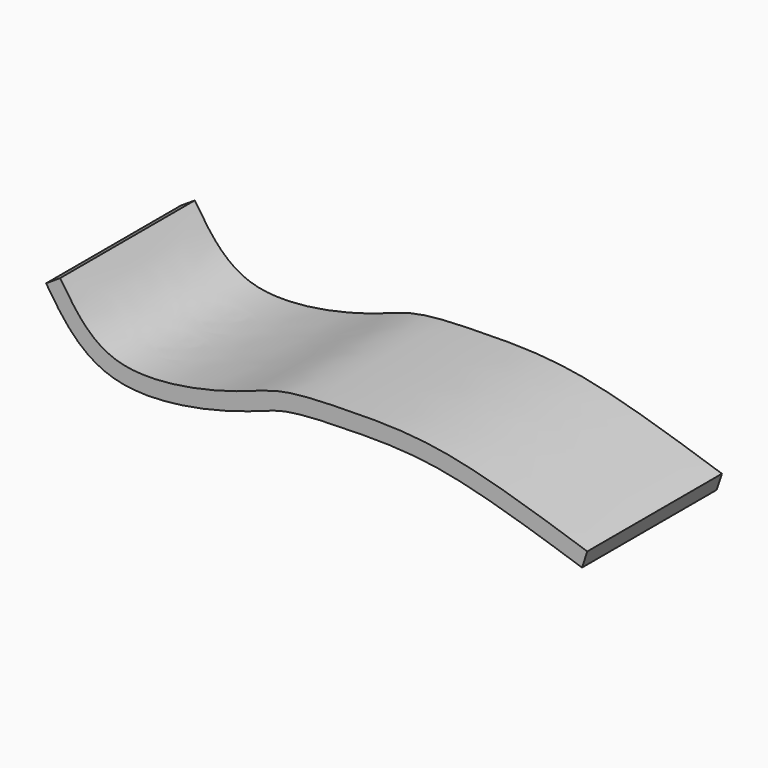
from build123d import *

# Parameters (mm, degrees)
F1_DEPTH = 30


# Not quite as in the source:
# - the dataset's text gives a spline's control points without its knots; the knots are read off the source's solid


with BuildPart() as f1:
    # F0 (on Front) → F1 (new body)
    with BuildSketch(Plane.XZ):
        with BuildLine():
            add(Edge.make_bspline(
                [(0, 0), (2.6760176861, -4.1090912765), (8.6109843066, -13.2223791643), (31.6156140644, -8.0154668369), (38.9230176312, -4.44082064), (51.783425309, -4.0415965154), (68.5152984785, -3.9207662334), (84.8401925941, -9.3146463612), (93.9818322659, -12.335119769)],
                knots=[0, 0, 0, 0, 0.1565314067, 0.3471608871, 0.4695561585, 0.6124947665, 0.7830042149, 1, 1, 1, 1], degree=3))
            Line((0, 0), (-2.5139018349, -1.6371614351))
            add(Edge.make_bspline(
                [(-2.5139018349, -1.6371614351), (-1.9796604679, -2.4575022542), (-0.8824950145, -4.1435116076), (0.9716962826, -6.681806788), (2.818494485, -8.6893851392), (4.557008715, -10.1358158216), (6.0060415743, -11.1092063701), (7.3415213838, -11.7998974719), (8.4850992129, -12.2638918131), (9.3820086025, -12.5650155809), (10.3070201286, -12.8131843436), (11.557238239, -13.0752296171), (13.1545045101, -13.2882162402), (15.1103366517, -13.3908370168), (17.7527257108, -13.3559807007), (21.0825413014, -13.0414284407), (24.9788204805, -12.3653086477), (28.0085066014, -11.6521555257), (30.2166637186, -11.0488210969), (31.7451800625, -10.5933469575), (33.119290683, -10.1496504012), (34.7509538884, -9.5877723837), (36.4769836834, -8.9563036794), (37.9277627865, -8.4589434042), (39.0494494043, -8.1389931547), (39.7663852968, -7.9682024182), (40.3766098683, -7.8468566795), (41.0225632514, -7.7333923842), (41.887025299, -7.6077797582), (43.0058157906, -7.482054254), (44.5913088845, -7.3455222102), (46.7249490736, -7.2266828348), (49.4553505745, -7.1438428112), (52.2981469692, -7.0863726415), (55.1415351216, -7.0513679222), (58.0217504556, -7.0809612374), (60.9631996142, -7.2074537938), (63.4895890714, -7.4223332941), (65.5709676375, -7.6772717752), (67.164506612, -7.9141125344), (68.7998566688, -8.2023954474), (71.0459002226, -8.6542298497), (73.959722197, -9.3354473137), (78.8117218745, -10.6357407606), (85.1614022918, -12.5803834941), (90.4076393103, -14.3136905098), (93.0406511874, -15.183659426)],
                knots=[0, 0, 0, 0, 0.03125, 0.0625, 0.09375, 0.109375, 0.125, 0.140625, 0.1484375, 0.15625, 0.1640625, 0.171875, 0.1875, 0.203125, 0.21875, 0.25, 0.28125, 0.3125, 0.328125, 0.34375, 0.359375, 0.375, 0.40625, 0.4375, 0.453125, 0.46875, 0.4765625, 0.484375, 0.5, 0.515625, 0.53125, 0.5625, 0.59375, 0.625, 0.65625, 0.6875, 0.71875, 0.75, 0.765625, 0.78125, 0.796875, 0.8125, 0.84375, 0.875, 0.9375, 1, 1, 1, 1], degree=3))
            Line((93.0406511874, -15.183659426), (93.9818322659, -12.335119769))
        make_face()
    extrude(amount=F1_DEPTH)


solid = f1.part
